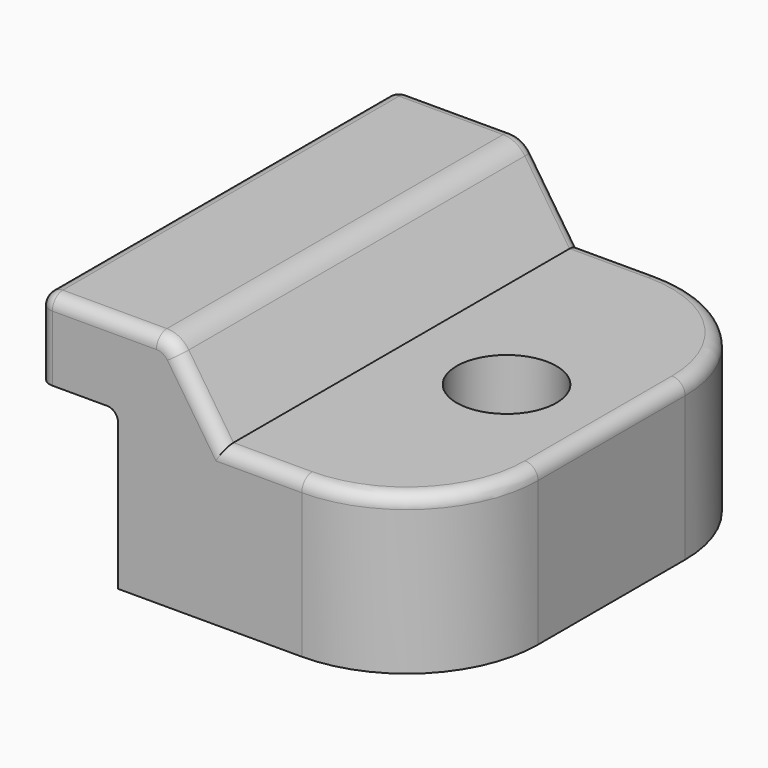
from build123d import *

# Parameters (mm, degrees)
F1_DEPTH = 17
F2_R     = 0.5
F3_R     = 1.9
F4_DEPTH = 25
F5_R     = 5
F6_R     = 0.5
F7_R     = 1
F8_R     = 0.49999


# Not quite as in the source:
# - a fillet or chamfer is up to 0.001 mm smaller than in the source, because OpenCascade refuses the exact size


with BuildPart() as f1:
    # F0 (on Front) → F1 (new body)
    with BuildSketch(Plane.XZ):
        with BuildLine():
            Line((-12, 0), (0, 0))
            Line((0, 0), (0, 5.58898558))
            ThreePointArc((0, 5.58898558), (0.1203833365, 5.8796166635), (0.41101442, 6))
            Line((0.41101442, 6), (3, 6))
            Line((3, 6), (3, 9))
            Line((3, 9), (-2, 9))
            Line((-2, 9), (-4, 6))
            Line((-4, 6), (-12, 6))
            Line((-12, 6), (-12, 0))
        make_face()
    extrude(amount=F1_DEPTH)

    # F2
    f2_edges = [f1.edges().sort_by_distance(p)[0] for p in [
        (3, -8.5, 9),
    ]]
    fillet(f2_edges, radius=F2_R)

    # F3 (on face) → F4 (cut)
    with BuildSketch(Plane.XY.offset(6)):
        with Locations((-8, -8.5)):
            Circle(F3_R)
    extrude(amount=-F4_DEPTH, mode=Mode.SUBTRACT)

    # F5
    f5_edges = [f1.edges().sort_by_distance(p)[0] for p in [
        (-12, -17, 3),
        (-12, 0, 3),
    ]]
    fillet(f5_edges, radius=F5_R)

    # F6
    f6_edges = [f1.edges().sort_by_distance(p)[0] for p in [
        (-10.535534, -15.535534, 6),
    ]]
    fillet(f6_edges, radius=F6_R)

    # F7
    f7_edges = [f1.edges().sort_by_distance(p)[0] for p in [
        (-2, -8.5, 9),
    ]]
    fillet(f7_edges, radius=F7_R)

    # F8 (radius 0.5 in the source; OpenCascade refuses exactly that, so slightly less here)
    f8_edges = [f1.edges().sort_by_distance(p)[0] for p in [
        (-3.148433, -17, 7.27735),
        (-3.148433, 0, 7.27735),
    ]]
    fillet(f8_edges, radius=F8_R)


with BuildPart() as f10_1:
    # F10: instance of F1
    add(f1.part.mirror(Plane(origin=(4, -8.5, 7.25), x_dir=(0, 1, 0), z_dir=(1, 0, 0))))


solid = f10_1.part
